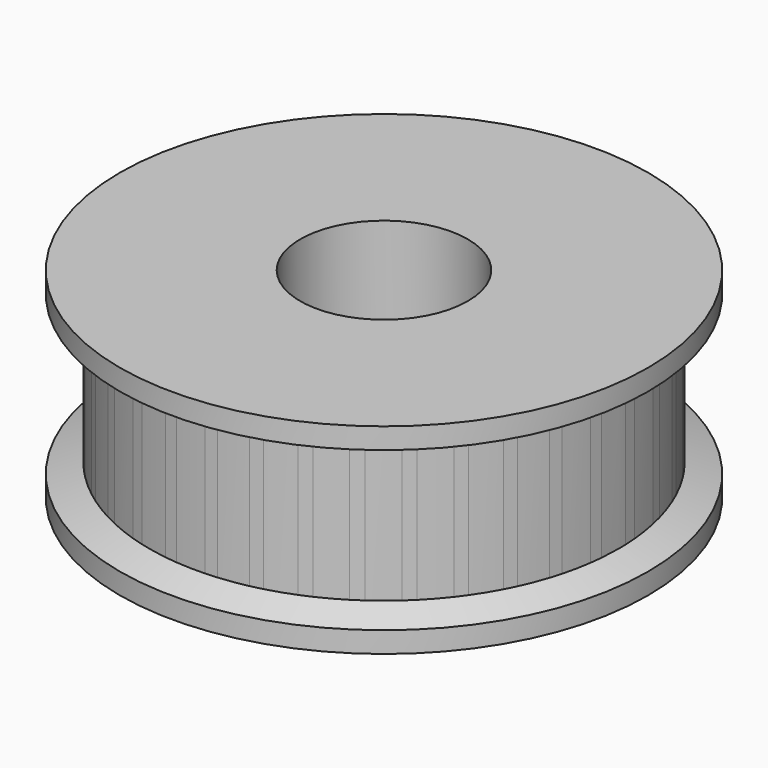
from build123d import *

# Parameters (mm, degrees)
F3_DEPTH = 4.5
F4_COUNT = 36
F7_R     = 4
F8_DEPTH = 50


# Not quite as in the source:
# - a feature names something its author has since deleted; it is built from what else it names


with BuildPart() as f3:
    # F2 (on Top) → F3 (new body, symmetric)
    with BuildSketch(Plane.XY):
        with BuildLine():
            Line((0.9112268782, 10.4153708779), (0.9765936853, 11.1625169015))
            ThreePointArc((0.9765936853, 11.1625169015), (0.4887620358, 11.1944910771), (0, 11.2051559026))
            ThreePointArc((0, 11.2051559026), (-0.2034888134, 11.2033080429), (-0.4069105114, 11.1977650733))
            ThreePointArc((-0.4069105114, 11.1977650733), (-0.6919765704, 11.1837689187), (-0.9765936853, 11.1625169015))
            Line((-0.9765936853, 11.1625169015), (-0.9112268782, 10.4153708779))
            Line((-0.9112268782, 10.4153708779), (0, 0))
            Line((0, 0), (0.9112268782, 10.4153708779))
        make_face()
    extrude(amount=F3_DEPTH, both=True)

    # F4: F3 ×36 about axis
    f4_axis = Axis((0, 0, 0), (0, 0, -1))


with BuildPart() as f3_1:
    add(f3.part)
    for i in range(1, F4_COUNT):
        add(f3.part.rotate(f4_axis, i * 360 / F4_COUNT))

    # F5 (on Front) → F6 (revolve)
    with BuildSketch(Plane.XZ):
        Polygon((12.6050714929, 4.5), (0, 4.5), (0, 2.717494719), (10.4551559026, 2.717494719), (12.6050714929, 3.5), align=None)
        Polygon((10.4551559026, -3.282505281), (0, -3.282505281), (0, -5.0650105621), (12.6050714929, -5.0650105621), (12.6050714929, -4.0650105621), align=None)
    revolve(axis=Axis((0, 0, 3.6087473595), (0, 0, 1)))

    # F7 (on Top) → F8 (cut, symmetric)
    with BuildSketch(Plane.XY):
        Circle(F7_R)
    extrude(amount=F8_DEPTH, both=True, mode=Mode.SUBTRACT)


solid = f3_1.part
